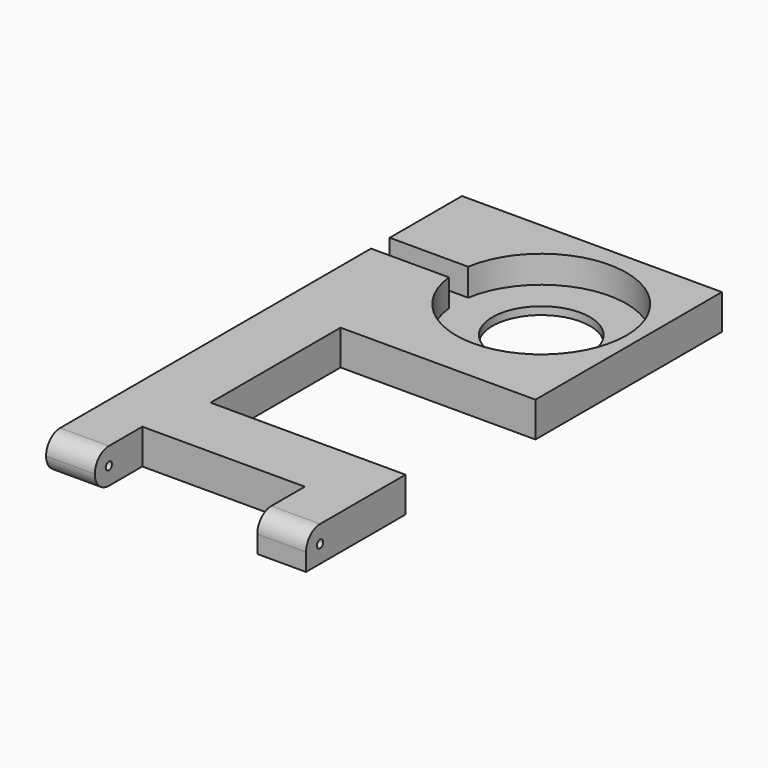
from build123d import *

# Parameters (mm, degrees)
F0_W      = 50.8
F0_H      = 101.6
F1_DEPTH  = 6.858
F2_R      = 16.637
F3_DEPTH  = 5.334
F4_R      = 9.525
F5_DEPTH  = 25.4
F6_W      = 31.75
F6_H      = 11.6078
F7_DEPTH  = 25.4
F8_W      = 38.1
F8_H      = 31.75
F9_DEPTH  = 25.4
F10_R     = 3.42899
F12_DEPTH = 5.334
F13_R     = 0.762
F14_DEPTH = 50.8


# Not quite as in the source:
# - a fillet or chamfer is up to 0.001 mm smaller than in the source, because OpenCascade refuses the exact size


with BuildPart() as f1:
    # F0 (on Top) → F1 (new body)
    with BuildSketch(Plane.XY):
        with Locations((6.0819597751, 21.255746996)):
            Rectangle(F0_W, F0_H)
    extrude(amount=F1_DEPTH)

    # F2 (on face) → F3 (cut)
    with BuildSketch(Plane.XY.offset(6.858)):
        with Locations((12.4319597751, 51.735746996)):
            Circle(F2_R)
    extrude(amount=-F3_DEPTH, mode=Mode.SUBTRACT)

    # F4 (on face) → F5 (cut)
    with BuildSketch(Plane.XY.offset(1.524)):
        with Locations((12.4319597751, 51.735746996)):
            Circle(F4_R)
    extrude(amount=-F5_DEPTH, mode=Mode.SUBTRACT)

    # F6 (on face) → F7 (cut)
    with BuildSketch(Plane.XY.offset(6.858)):
        with Locations((6.0819597751, -23.740353004)):
            Rectangle(F6_W, F6_H)
    extrude(amount=-F7_DEPTH, mode=Mode.SUBTRACT)

    # F8 (on face) → F9 (cut)
    with BuildSketch(Plane.XY.offset(6.858)):
        with Locations((12.4319597751, 10.638546996)):
            Rectangle(F8_W, F8_H)
    extrude(amount=-F9_DEPTH, mode=Mode.SUBTRACT)

    # F10 (radius 3.429 in the source; OpenCascade refuses exactly that, so slightly less here)
    f10_edges = [f1.edges().sort_by_distance(p)[0] for p in [
        (-14.55554, -29.544253, 6.858),
        (26.71946, -29.544253, 6.858),
        (-14.55554, -29.544253, 0),
    ]]
    fillet(f10_edges, radius=F10_R)

    # F11 (on face) → F12 (cut)
    with BuildSketch(Plane.XY.offset(6.858)):
        with BuildLine():
            Line((-3.9898817782, 54.402746996), (-19.3180402249, 54.402746996))
            Line((-19.3180402249, 54.402746996), (-19.3180402249, 49.830746996))
            Line((-19.3180402249, 49.830746996), (-4.0956154857, 49.830746996))
            ThreePointArc((-4.0956154857, 49.830746996), (-4.2005930385, 52.1203973622), (-3.9898817782, 54.402746996))
        make_face()
    extrude(amount=-F12_DEPTH, mode=Mode.SUBTRACT)

    # F13 (on face) → F14 (cut)
    with BuildSketch(Plane(origin=(-19.3180402249, 0, 0), x_dir=(0, -1, 0), z_dir=(-1, 0, 0))):
        with Locations((26.115253004, 3.429)):
            Circle(F13_R)
    extrude(amount=-F14_DEPTH, mode=Mode.SUBTRACT)


solid = f1.part
